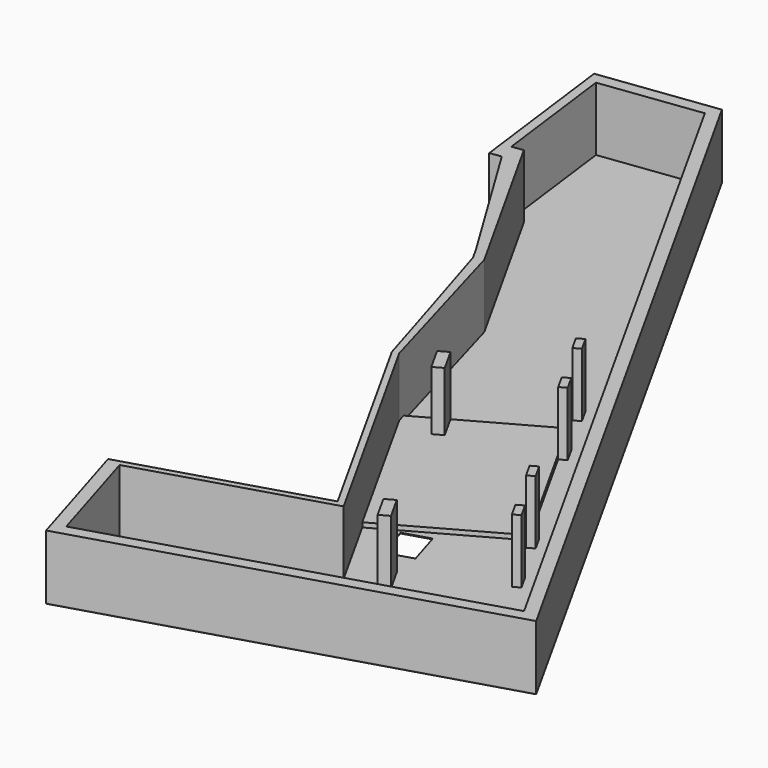
from build123d import *

# Parameters (mm, degrees)
F3_DEPTH  = 2100
F5_DEPTH  = 25
F7_DEPTH  = 2100
F9_DEPTH  = 150
F11_DEPTH = 25.001


# Not quite as in the source:
# - ends of sketch curves that miss each other by under 0.0002 mm in the source are joined


with BuildPart() as f3:
    # F2 (on Top) → F3 (new body)
    with BuildSketch(Plane.XY):
        Polygon((52902.0595629306, 50434.1230428591), (54145.32292, 46326.602018), (54431.4219269024, 46413.1983883223), (67150.915474, 50263.131268), (53075.201891, 75510.702684), (49253.5741891713, 75020.4629237414), (49304.213105, 74623.774346), (49909.660074, 69880.902321), (50281.682258, 69933.639978), (53000.597675, 65468.812402), (53225.019852, 65066.306629), (54325.972768, 61474.063518), (54760.522861, 60038.387295), (54874.022799, 59663.37285), (58991.897227, 52278.191447), (57604.002801, 51858.903346), (53909.97748, 50739.1999), align=None)
        Polygon((54412.25928, 46825.31334), (53342.81403, 50358.57026), (59287.509616, 52158.706562), (55070.827017, 59721.094989), (53523.858293, 65159.740021), (50504.389213421, 70561.8996273451), (50131.257661, 70514.151722), (49601.798244, 74661.762303), (52857.629236, 75079.514646), (66559.719817, 50502.109853), align=None, mode=Mode.SUBTRACT)
    extrude(amount=F3_DEPTH)


with BuildPart() as f5:
    # F4 (on Top) → F5 (new body)
    with BuildSketch(Plane.XY):
        Polygon((54760.522861, 60038.387295), (54874.022799, 59663.37285), (58991.897227, 52278.191447), (57604.002801, 51858.903346), (53909.97748, 50739.1999), (52902.0595629306, 50434.1230428591), (54145.32292, 46326.602018), (67150.915474, 50263.131268), (53075.201891, 75510.702684), (49253.5741891713, 75020.4629237414), (49304.213105, 74623.774346), (49909.660074, 69880.902321), (50281.682258, 69933.639978), (53000.597675, 65468.812402), (53225.019852, 65066.306629), (54325.972768, 61474.063518), align=None)
    extrude(amount=-F5_DEPTH)

    # F6 (on Top) → F7 (join)
    with BuildSketch(Plane.XY):
        Polygon((63167.175561, 54636.370609), (62899.326908, 55116.742443), (62680.976074, 54994.993056), (62948.824727, 54514.621222), align=None)
        Polygon((61606.57177, 56922.149305), (61874.420423, 56441.777471), (62092.771256, 56563.526859), (61824.922604, 57043.898693), align=None)
        Polygon((60131.75578, 53293.714353), (59826.064613, 53123.26521), (60264.362406, 52337.202212), (60570.053573, 52507.651355), align=None)
        Polygon((56498.652366, 59810.307311), (56060.354571, 60596.370312), (55754.663404, 60425.921169), (56192.961199, 59639.858168), align=None)
        Polygon((59393.320264, 61405.457583), (59174.969431, 61283.708196), (59442.818085, 60803.336359), (59661.168918, 60925.085747), align=None)
        Polygon((58586.764842, 62852.241589), (58318.916189, 63332.613423), (58100.565355, 63210.864035), (58368.414008, 62730.492201), align=None)
    extrude(amount=F7_DEPTH)

    # F10 (on face) → F11 (cut, through all)
    with BuildSketch(Plane.XY):
        Polygon((59168.735458, 53933.31513), (60028.231633, 54193.415485), (59680.654869, 55341.975624), (58821.158694, 55081.875269), align=None)
    extrude(amount=-F11_DEPTH, mode=Mode.SUBTRACT)


with BuildPart() as f9:
    # F8 (on Top) → F9 (new body)
    with BuildSketch(Plane.XY):
        Polygon((58728.797232615, 62084.088870835), (56060.354571, 60596.370312), (56498.652366, 59810.307311), (56192.961199, 59639.858168), (55754.663404, 60425.921169), (54991.3996931603, 60000.3359416475), (55070.827017, 59721.094989), (55102.8168784927, 59663.7229310719), (57874.844064254, 54692.2445670372), (58565.3824039826, 55077.2791403316), (61670.1839855803, 56808.2778988538), align=None)
    extrude(amount=F9_DEPTH)


solid = Compound([f3.part, f5.part, f9.part])
